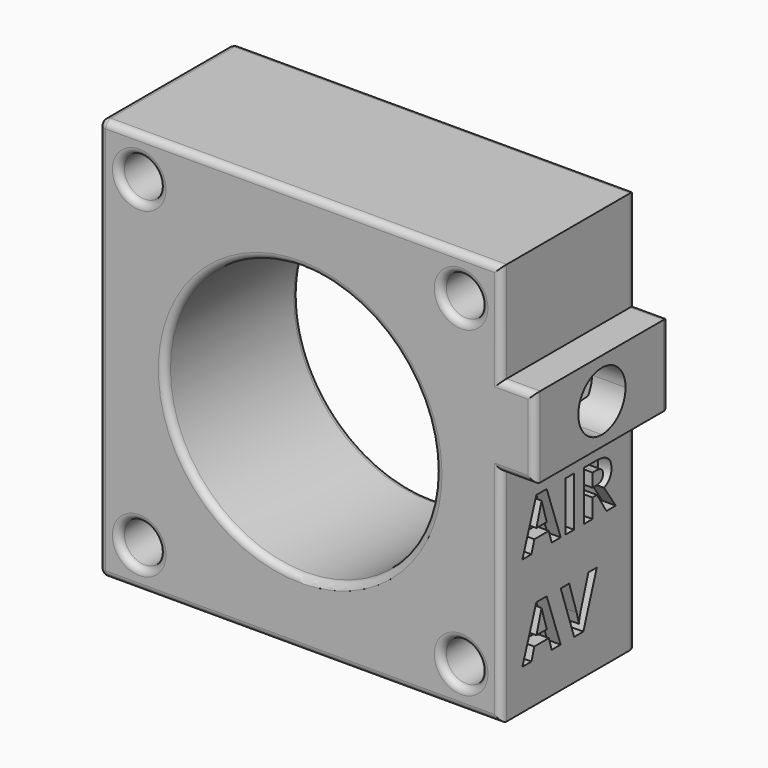
from build123d import *

# Parameters (mm, degrees)
F0_W          = 60
F0_H          = 60
F0_R          = 3
F0_R_2        = 20.15
F1_DEPTH      = 25
F4_W          = 3.5
F4_H          = 20
F5_DEPTH      = 50
F6_W          = 25
F6_H          = 12
F6_W_2        = 20
F6_H_2        = 4.9497474683
F7_DEPTH      = 5
F9_DEPTH      = 7
F10_R         = 1
F11_TEXT_SIZE = 10.353239486
F12_DEPTH     = 2


# Not quite as in the source:
# - Text() gives the source's letters only with a copy of the font that has no kerning and outlines rounded to 1/6400 em; it was checked with that copy


with BuildPart() as f1:
    # F0 (on Front) → F1 (new body)
    with BuildSketch(Plane.XZ):
        Rectangle(F0_W, F0_H)
        with Locations((-24, -24)):
            Circle(F0_R, mode=Mode.SUBTRACT)
        with Locations((24, -24)):
            Circle(F0_R, mode=Mode.SUBTRACT)
        with Locations((-24, 24)):
            Circle(F0_R, mode=Mode.SUBTRACT)
        Circle(F0_R_2, mode=Mode.SUBTRACT)
        with Locations((24, 24)):
            Circle(F0_R, mode=Mode.SUBTRACT)
    extrude(amount=F1_DEPTH)

    # F4 (on face) → F5 (cut)
    with BuildSketch(Plane(origin=(30, 0, 30), x_dir=(0.7071067812, 0, -0.7071067812), z_dir=(0.7071067812, 0, 0.7071067812))):
        with Locations((14.8124283052, -12.5)):
            Rectangle(F4_W, F4_H)
    extrude(amount=-F5_DEPTH, mode=Mode.SUBTRACT)

    # F6 (on face) → F7 (join)
    with BuildSketch(Plane.YZ.offset(30)):
        with Locations((-12.5, 9)):
            Rectangle(F6_W, F6_H)
        with Locations((-12.5, 9.0520629991)):
            Rectangle(F6_W_2, F6_H_2, mode=Mode.SUBTRACT)
        with Locations((-12.5, 9.0520629991)):
            Rectangle(F6_W_2, F6_H_2)
    extrude(amount=F7_DEPTH)

    # F8 (on face) → F9 (cut)
    with BuildSketch(Plane.YZ.offset(35)):
        with BuildLine():
            Line((-12.5, 4.6), (-12.5, 9))
            Line((-12.5, 9), (-16.9, 9))
            ThreePointArc((-16.9, 9), (-15.6112698372, 5.8887301628), (-12.5, 4.6))
        make_face()
        with BuildLine():
            Line((-12.5, 9), (-12.5, 13.4))
            ThreePointArc((-12.5, 13.4), (-15.6112698372, 12.1112698372), (-16.9, 9))
            Line((-16.9, 9), (-12.5, 9))
        make_face()
        with BuildLine():
            ThreePointArc((-8.1, 9), (-9.3887301628, 12.1112698372), (-12.5, 13.4))
            Line((-12.5, 13.4), (-12.5, 9))
            Line((-12.5, 9), (-8.1, 9))
        make_face()
        with BuildLine():
            Line((-8.1, 9), (-12.5, 9))
            Line((-12.5, 9), (-12.5, 4.6))
            ThreePointArc((-12.5, 4.6), (-9.3887301628, 5.8887301628), (-8.1, 9))
        make_face()
    extrude(amount=-F9_DEPTH, mode=Mode.SUBTRACT)

    # F10
    f10_edges = [f1.edges().sort_by_distance(p)[0] for p in [
        (-30, -12.5, 30),
        (-30, -12.5, -30),
        (-30, 0, 0),
        (-30, -25, 0),
        (0, 0, -30),
        (30, 0, -13.5),
        (32.5, 0, 3),
        (35, 0, 9),
        (32.5, 0, 15),
        (30, 0, 22.5),
        (0, 0, 30),
        (-27, 0, -24),
        (21, 0, -24),
        (-27, 0, 24),
        (-20.15, 0, 0),
        (21, 0, 24),
        (0, -25, -30),
        (30, -25, -13.5),
        (32.5, -25, 3),
        (35, -25, 9),
        (32.5, -25, 15),
        (30, -25, 22.5),
        (0, -25, 30),
        (-27, -25, -24),
        (21, -25, -24),
        (-27, -25, 24),
        (-20.15, -25, 0),
        (21, -25, 24),
    ]]
    fillet(f10_edges, radius=F10_R)

    # F11 (on face) → F12 (cut)
    with BuildSketch(Plane.YZ.offset(30)):
        with Locations((-21.0774708539, -9.9314050749)):
            Text('AIR', F11_TEXT_SIZE, font='Open Sans', font_style=FontStyle.BOLD, text_align=(TextAlign.LEFT, TextAlign.BOTTOM))
        with Locations((-21.0774708539, -24.0118107758)):
            Text('AV', F11_TEXT_SIZE, font='Open Sans', font_style=FontStyle.BOLD, text_align=(TextAlign.LEFT, TextAlign.BOTTOM))
    extrude(amount=-F12_DEPTH, mode=Mode.SUBTRACT)


solid = f1.part
